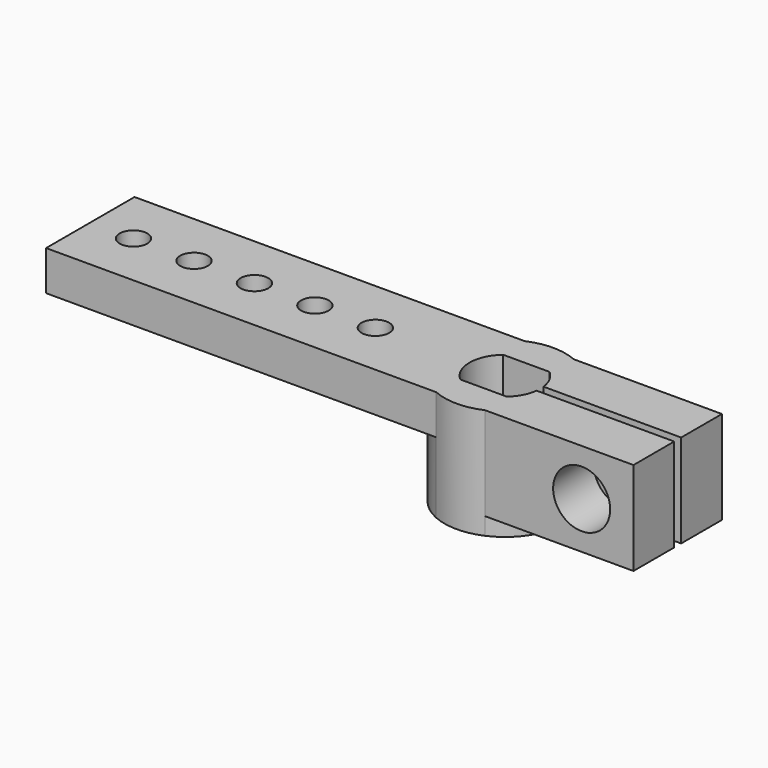
from build123d import *
from build123d import SkipClean  # not in build123d's __all__

# Parameters (mm, degrees)
F0_R     = 0.8
F1_DEPTH = 6.4
F2_DEPTH = 1
F3_DEPTH = 4.1
F4_W     = 0.5
F4_H     = 15
F5_DEPTH = 25
F7_D     = 3.3
F7_DEPTH = 3.2
F7_TIP   = 0.9914200214
F8_D     = 2.4
F8_DEPTH = 3.5
F8_TIP   = 0.7210327428


with BuildPart() as f1:
    # F0 (on Top) → F1 (new body)
    with BuildSketch(Plane.XY):
        with BuildLine():
            Line((-24, -3.2), (-1.4177446879, -3.2))
            ThreePointArc((-1.4177446879, -3.2), (-2.4227036384, -2.5259665636), (-3.1380726569, -1.55))
            ThreePointArc((-3.1380726569, -1.55), (-3.5, 0), (-3.1380726569, 1.55))
            ThreePointArc((-3.1380726569, 1.55), (-2.4227036384, 2.5259665636), (-1.4177446879, 3.2))
            Line((-1.4177446879, 3.2), (-24, 3.2))
            Line((-24, 3.2), (-24, -3.2))
        make_face()
        with Locations((-21.5, 0)):
            Circle(F0_R, mode=Mode.SUBTRACT)
        with Locations((-18, 0)):
            Circle(F0_R, mode=Mode.SUBTRACT)
        with Locations((-14.5, 0)):
            Circle(F0_R, mode=Mode.SUBTRACT)
        with Locations((-11, 0)):
            Circle(F0_R, mode=Mode.SUBTRACT)
        with Locations((-7.5, 0)):
            Circle(F0_R, mode=Mode.SUBTRACT)
        with BuildLine():
            Line((-3.1380726569, -1.55), (-1.3416407865, -1.55))
            ThreePointArc((-1.3416407865, -1.55), (-2.05, 0), (-1.3416407865, 1.55))
            Line((-1.3416407865, 1.55), (-3.1380726569, 1.55))
            ThreePointArc((-3.1380726569, 1.55), (-3.5, 0), (-3.1380726569, -1.55))
        make_face()
        with BuildLine():
            ThreePointArc((1.4177446879, -3.2), (2.4227036384, -2.5259665636), (3.1380726569, -1.55))
            Line((3.1380726569, -1.55), (1.3416407865, -1.55))
            ThreePointArc((1.3416407865, -1.55), (0, -2.05), (-1.3416407865, -1.55))
            Line((-1.3416407865, -1.55), (-3.1380726569, -1.55))
            ThreePointArc((-3.1380726569, -1.55), (-2.4227036384, -2.5259665636), (-1.4177446879, -3.2))
            Line((-1.4177446879, -3.2), (1.4177446879, -3.2))
        make_face()
        with BuildLine():
            Line((1.3416407865, 1.55), (3.1380726569, 1.55))
            ThreePointArc((3.1380726569, 1.55), (2.4227036384, 2.5259665636), (1.4177446879, 3.2))
            Line((1.4177446879, 3.2), (-1.4177446879, 3.2))
            ThreePointArc((-1.4177446879, 3.2), (-2.4227036384, 2.5259665636), (-3.1380726569, 1.55))
            Line((-3.1380726569, 1.55), (-1.3416407865, 1.55))
            ThreePointArc((-1.3416407865, 1.55), (0, 2.05), (1.3416407865, 1.55))
        make_face()
        with BuildLine():
            ThreePointArc((1.3416407865, 1.55), (0, 2.05), (-1.3416407865, 1.55))
            Line((-1.3416407865, 1.55), (1.3416407865, 1.55))
        make_face()
        with BuildLine():
            ThreePointArc((-1.3416407865, -1.55), (0, -2.05), (1.3416407865, -1.55))
            Line((1.3416407865, -1.55), (-1.3416407865, -1.55))
        make_face()
        with BuildLine():
            Line((1.3416407865, -1.55), (3.1380726569, -1.55))
            ThreePointArc((3.1380726569, -1.55), (3.4083173487, -0.7958472532), (3.5, 0))
            ThreePointArc((3.5, 0), (3.4083173487, 0.7958472532), (3.1380726569, 1.55))
            Line((3.1380726569, 1.55), (1.3416407865, 1.55))
            ThreePointArc((1.3416407865, 1.55), (1.864519189, 0.8520963524), (2.05, 0))
            ThreePointArc((2.05, 0), (1.864519189, -0.8520963524), (1.3416407865, -1.55))
        make_face()
        with BuildLine():
            ThreePointArc((3.5, 0), (3.4083173487, -0.7958472532), (3.1380726569, -1.55))
            ThreePointArc((3.1380726569, -1.55), (2.4227036384, -2.5259665636), (1.4177446879, -3.2))
            Line((1.4177446879, -3.2), (10, -3.2))
            Line((10, -3.2), (10, 3.2))
            Line((10, 3.2), (1.4177446879, 3.2))
            ThreePointArc((1.4177446879, 3.2), (2.4227036384, 2.5259665636), (3.1380726569, 1.55))
            ThreePointArc((3.1380726569, 1.55), (3.4083173487, 0.7958472532), (3.5, 0))
        make_face()
        with BuildLine():
            ThreePointArc((-1.4177446879, -3.2), (0, -3.5), (1.4177446879, -3.2))
            Line((1.4177446879, -3.2), (-1.4177446879, -3.2))
        make_face()
        with BuildLine():
            Line((-1.4177446879, 3.2), (1.4177446879, 3.2))
            ThreePointArc((1.4177446879, 3.2), (0, 3.5), (-1.4177446879, 3.2))
        make_face()
    extrude(amount=F1_DEPTH)

    # F0 (on Top) → F2 (cut)
    with BuildSketch(Plane.XY):
        with BuildLine():
            ThreePointArc((3.5, 0), (3.4083173487, -0.7958472532), (3.1380726569, -1.55))
            ThreePointArc((3.1380726569, -1.55), (2.4227036384, -2.5259665636), (1.4177446879, -3.2))
            Line((1.4177446879, -3.2), (10, -3.2))
            Line((10, -3.2), (10, 3.2))
            Line((10, 3.2), (1.4177446879, 3.2))
            ThreePointArc((1.4177446879, 3.2), (2.4227036384, 2.5259665636), (3.1380726569, 1.55))
            ThreePointArc((3.1380726569, 1.55), (3.4083173487, 0.7958472532), (3.5, 0))
        make_face()
    with SkipClean():  # cleaning this boolean's faces spoils the solid; the shape is the same uncleaned
        extrude(amount=F2_DEPTH, mode=Mode.SUBTRACT)

    # F0 (on Top) → F3 (cut)
    with BuildSketch(Plane.XY):
        with BuildLine():
            Line((-24, -3.2), (-1.4177446879, -3.2))
            ThreePointArc((-1.4177446879, -3.2), (-2.4227036384, -2.5259665636), (-3.1380726569, -1.55))
            ThreePointArc((-3.1380726569, -1.55), (-3.5, 0), (-3.1380726569, 1.55))
            ThreePointArc((-3.1380726569, 1.55), (-2.4227036384, 2.5259665636), (-1.4177446879, 3.2))
            Line((-1.4177446879, 3.2), (-24, 3.2))
            Line((-24, 3.2), (-24, -3.2))
        make_face()
        with Locations((-21.5, 0)):
            Circle(F0_R, mode=Mode.SUBTRACT)
        with Locations((-18, 0)):
            Circle(F0_R, mode=Mode.SUBTRACT)
        with Locations((-14.5, 0)):
            Circle(F0_R, mode=Mode.SUBTRACT)
        with Locations((-11, 0)):
            Circle(F0_R, mode=Mode.SUBTRACT)
        with Locations((-7.5, 0)):
            Circle(F0_R, mode=Mode.SUBTRACT)
    extrude(amount=F3_DEPTH, mode=Mode.SUBTRACT)

    # F4 (on Right) → F5 (cut)
    with BuildSketch(Plane.YZ):
        Rectangle(F4_W, F4_H)
    extrude(amount=F5_DEPTH, mode=Mode.SUBTRACT)

    # F7 (one way)
    with BuildSketch(Plane(origin=(0, 0, 0), x_dir=(1, 0, 0), z_dir=(0, 1, 0))):
        with Locations((7, -3.7)):
            Circle(F7_D / 2)
    extrude(amount=-F7_DEPTH, mode=Mode.SUBTRACT)
    with Locations(Plane(origin=(0, 0, 0), x_dir=(1, 0, 0), z_dir=(0, 1, 0))):
        with Locations((7, -3.7)):
            with Locations((0, 0, -(F7_DEPTH + F7_TIP / 2))):  # 118° drill point
                Cone(0, F7_D / 2, F7_TIP, mode=Mode.SUBTRACT)

    # F8
    with Locations(Plane.XZ):
        with Locations((7, 3.7)):
            Hole(F8_D / 2, depth=F8_DEPTH)
            with Locations((0, 0, -(F8_DEPTH + F8_TIP / 2))):  # 118° drill point
                Cone(0, F8_D / 2, F8_TIP, mode=Mode.SUBTRACT)


solid = f1.part
